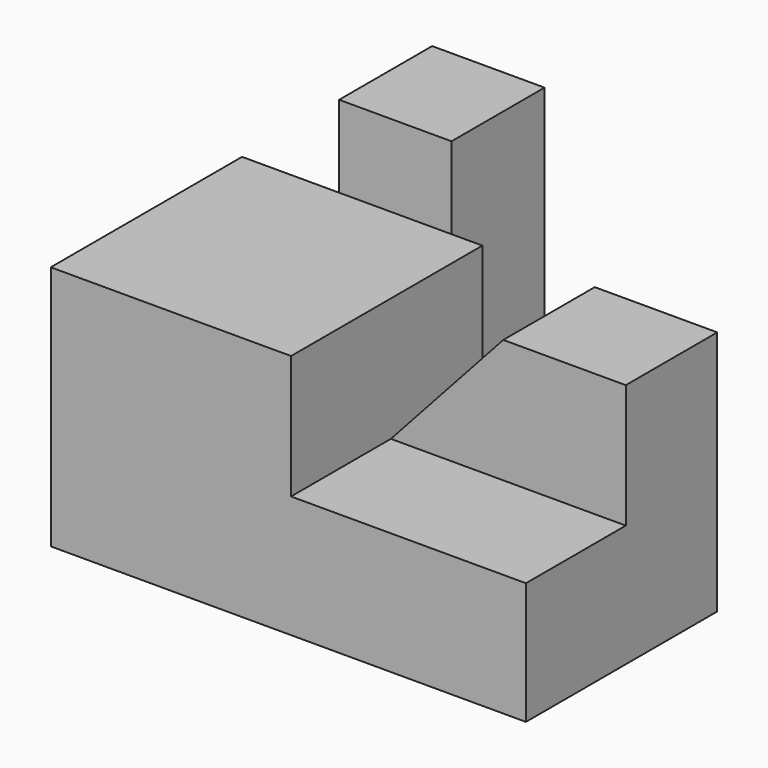
from build123d import *

# Parameters (mm, degrees)
F0_W     = 15.3924
F0_H     = 8.001
F1_DEPTH = 15.6718
F3_DEPTH = 7.493
F5_DEPTH = 7.9502
F7_DEPTH = 7.62


with BuildPart() as f1:
    # F0 (on Front) → F1 (new body)
    with BuildSketch(Plane.XZ):
        with Locations((23.4442, 4.0005)):
            Rectangle(F0_W, F0_H)
        Polygon((0, 16.1036), (0, 0), (15.748, 0), (15.748, 8.001), (15.748, 16.1036), align=None)
    extrude(amount=F1_DEPTH)

    # F2 (on face) → F3 (join)
    with BuildSketch(Plane(origin=(0, 0, 0), x_dir=(-1, 0, 0), z_dir=(0, 1, 0))):
        Polygon((-31.1404, 16.1036), (-31.1404, 8.001), (-15.748, 8.001), (-23.113546893, 16.1036), align=None)
    extrude(amount=-F3_DEPTH)

    # F4 (on face) → F5 (join)
    with BuildSketch(Plane(origin=(0, 0, 0), x_dir=(-1, 0, 0), z_dir=(0, 1, 0))):
        Polygon((-7.366, 0), (0, 0), (0, 7.7724), align=None)
    extrude(amount=F5_DEPTH)

    # F6 (on face) → F7 (join)
    with BuildSketch(Plane(origin=(0, 7.9502, 0), x_dir=(-1, 0, 0), z_dir=(0, 1, 0))):
        Polygon((-7.366, 0), (0, 0), (0, 7.7724), align=None)
        Polygon((-7.366, 16.163635999), (-7.366, 0), (0, 7.7724), (0, 16.163635999), align=None)
    extrude(amount=F7_DEPTH)


solid = f1.part
